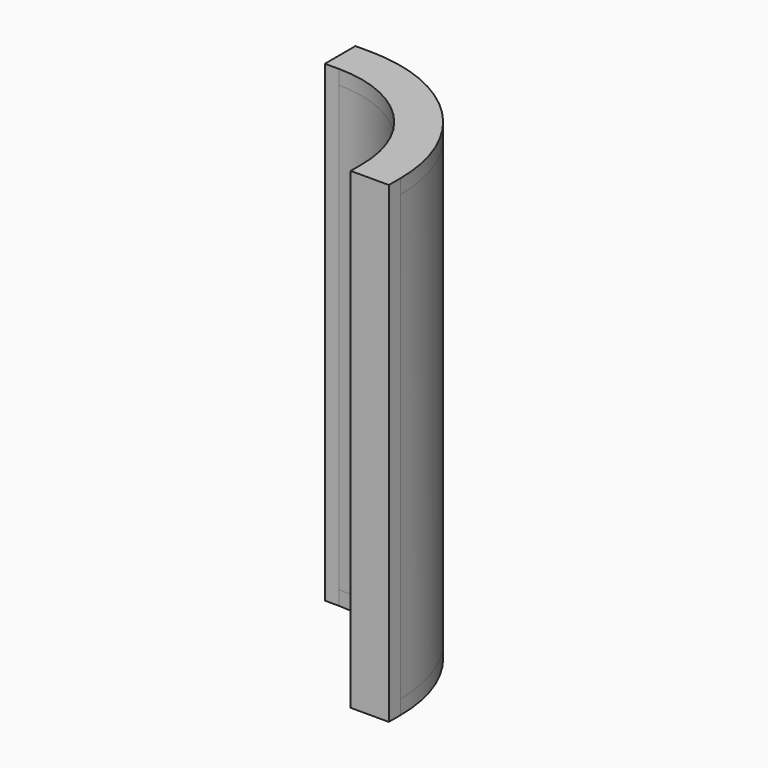
from build123d import *

# Parameters (mm, degrees)
F1_DEPTH = 2.38125
F0_W     = 6.35
F0_H     = 2.38125
F0_W_2   = 2.38125
F0_H_2   = 6.35
F2_DEPTH = 76.2
F3_W     = 6.35
F3_H     = 2.38125
F3_W_2   = 2.38125
F3_H_2   = 6.35
F4_DEPTH = 2.38125
F5_DEPTH = 73.81875


# Not quite as in the source:
# - a length typed as a fraction of an inch, garbled in the dataset ("3 / 203.2 mm" for 3/8 in), is restored
# - a feature names something its author has since deleted; it is built from what else it names


with BuildPart() as f1:
    # F0 (on Top) → F1 (new body)
    with BuildSketch(Plane.XY):
        with BuildLine():
            ThreePointArc((0, 19.05), (13.4703841816, 13.4703841816), (19.05, 0))
            Line((19.05, 0), (25.4, 0))
            ThreePointArc((25.4, 0), (17.9605122421, 17.9605122421), (0, 25.4))
            Line((0, 25.4), (0, 19.05))
        make_face()
    extrude(amount=F1_DEPTH)

    # F0 (on Top) → F2 (join)
    with BuildSketch(Plane.XY):
        with Locations((22.225, -1.190625)):
            Rectangle(F0_W, F0_H)
        with Locations((-1.190625, 22.225)):
            Rectangle(F0_W_2, F0_H_2)
    extrude(amount=F2_DEPTH)

    # F3 (on face) → F4 (join)
    with BuildSketch(Plane.XY.offset(76.2)):
        with Locations((22.225, -1.190625)):
            Rectangle(F3_W, F3_H)
        with BuildLine():
            ThreePointArc((0, 19.05), (13.4703841816, 13.4703841816), (19.05, 0))
            Line((19.05, 0), (25.4, 0))
            ThreePointArc((25.4, 0), (17.9605122421, 17.9605122421), (0, 25.4))
            Line((0, 25.4), (0, 19.05))
        make_face()
        with Locations((-1.190625, 22.225)):
            Rectangle(F3_W_2, F3_H_2)
    extrude(amount=F4_DEPTH)


with BuildPart() as f5:
    # F5 (new): a face of the model
    f5_faces = [f1.part.faces().sort_by_distance(p)[0] for p in [
        (14.2451252874, 14.2451252874, 2.38125),
    ]]
    extrude(f5_faces, amount=F5_DEPTH)


solid = Compound([f1.part, f5.part])
